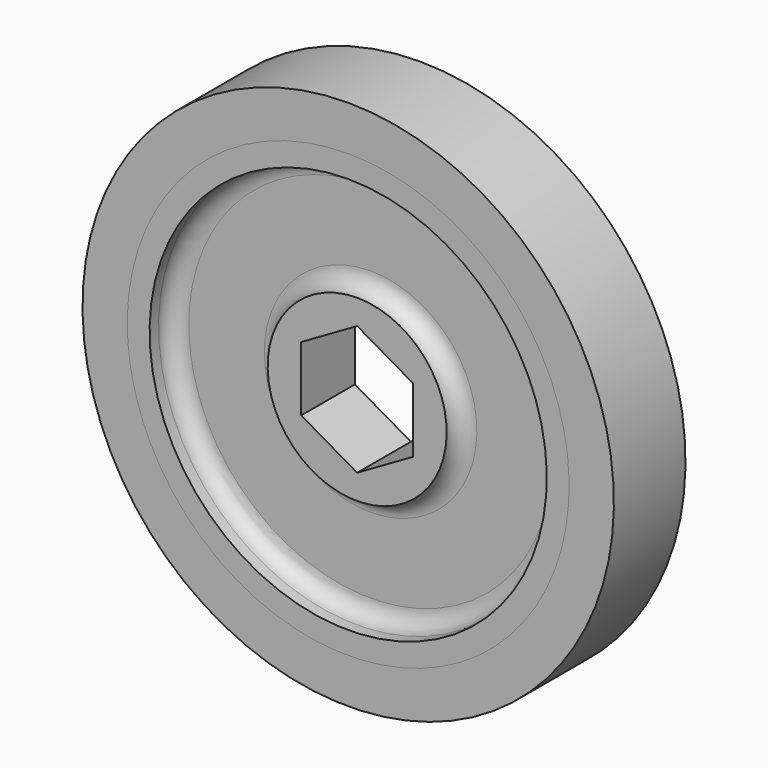
from build123d import *

# Parameters (mm, degrees)
F2_R     = 1.90499
F4_DEPTH = 7.62


# Not quite as in the source:
# - a fillet or chamfer is up to 0.001 mm smaller than in the source, because OpenCascade refuses the exact size


with BuildPart() as f1:
    # F0 (on Right) → F1 (revolve)
    with BuildSketch(Plane.YZ):
        Polygon((-3.81, 10.16), (-3.81, 0), (3.81, 0), (3.81, 10.16), (1.905, 10.16), (1.905, 22.5425), (5.08, 22.5425), (5.08, 25.0825), (2.54, 25.0825), (2.54, 27.6225), (-2.54, 27.6225), (-2.54, 25.0825), (-5.08, 25.0825), (-5.08, 22.5425), (-1.905, 22.5425), (-1.905, 10.16), align=None)
    revolve(axis=Axis((0, 0, 0), (0, 1, 0)))

    # F2 (radius 1.905 in the source; OpenCascade refuses exactly that, so slightly less here)
    f2_edges = [f1.edges().sort_by_distance(p)[0] for p in [
        (0, 1.905, -10.16),
        (0, 1.905, -22.5425),
        (0, -1.905, -10.16),
        (0, -1.905, -22.5425),
    ]]
    fillet(f2_edges, radius=F2_R)

    # F3 (on face) → F4 (cut, through all)
    with BuildSketch(Plane.XZ.offset(3.81)):
        Polygon((6.35, -3.6661742094), (6.35, 3.6661742094), (0, 7.3323484187), (-6.35, 3.6661742094), (-6.35, -3.6661742094), (0, -7.3323484187), align=None)
    extrude(amount=-F4_DEPTH, mode=Mode.SUBTRACT)


with BuildPart() as f6:
    # F5 (on Right) → F6 (revolve)
    with BuildSketch(Plane.YZ):
        Polygon((-5.08, 30.1625), (-5.08, 25.0825), (-2.54, 25.0825), (-2.54, 27.6225), (2.54, 27.6225), (2.54, 25.0825), (5.08, 25.0825), (5.08, 30.1625), align=None)
    revolve(axis=Axis((0, 0, 0), (0, 1, 0)))


solid = Compound([f1.part, f6.part])
